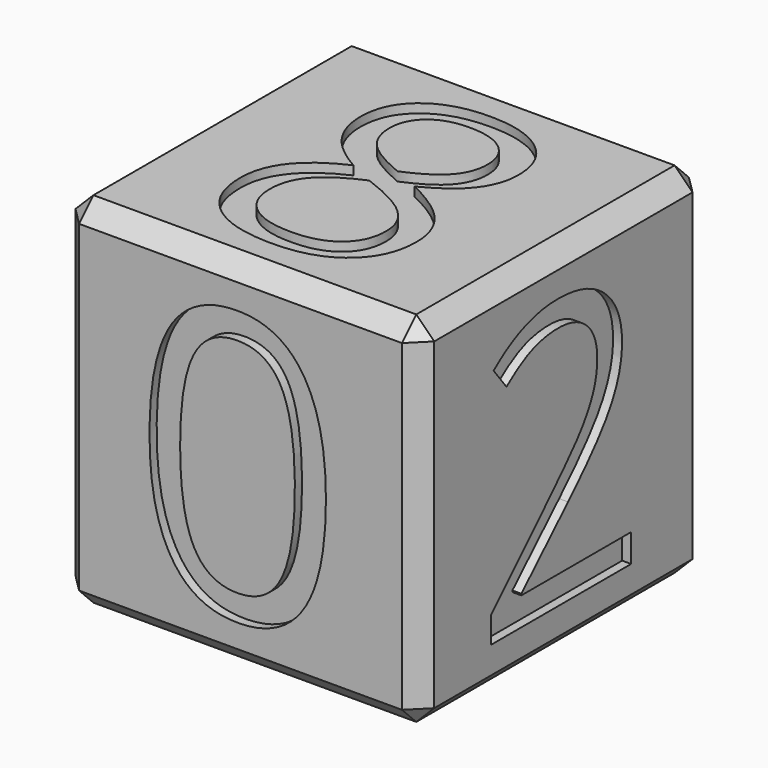
from build123d import *

# Parameters (mm, degrees)
F0_W          = 50.8
F0_H          = 50.8
F1_DEPTH      = 25.4
F1_DEPTH_BACK = 25.4
F2_SIZE       = 2.54
F3_TEXT_SIZE  = 52.9166666667
F4_DEPTH      = 1.27
F5_TEXT_SIZE  = 52.9166666667
F6_DEPTH      = 1.27
F7_TEXT_SIZE  = 52.9166666667
F8_DEPTH      = 1.27
F9_TEXT_SIZE  = 52.9166666667
F10_DEPTH     = 1.27
F11_TEXT_SIZE = 52.9166666667
F12_DEPTH     = 1.27
F13_TEXT_SIZE = 52.9166666667
F14_DEPTH     = 1.27


# Not quite as in the source:
# - Text() gives the source's letters only with a copy of the font that has no kerning and outlines rounded to 1/6400 em; it was checked with that copy


with BuildPart() as f1:
    # F0 (on Top) → F1 (new body, two sides)
    with BuildSketch(Plane.XY) as f1_sk:
        Rectangle(F0_W, F0_H)
    extrude(amount=F1_DEPTH)
    extrude(f1_sk.sketch, amount=-F1_DEPTH_BACK)

    # F2
    f2_edges = [f1.edges().sort_by_distance(p)[0] for p in [
        (0, 25.4, 25.4),
        (-25.4, 25.4, 0),
        (0, 25.4, -25.4),
        (25.4, 25.4, 0),
        (25.4, 0, 25.4),
        (-25.4, 0, 25.4),
        (0, -25.4, 25.4),
        (25.4, -25.4, 0),
        (25.4, 0, -25.4),
        (-25.4, 0, -25.4),
        (0, -25.4, -25.4),
        (-25.4, -25.4, 0),
    ]]
    chamfer(f2_edges, length=F2_SIZE)

    # F3 (on face) → F4 (cut)
    with BuildSketch(Plane.XZ.offset(25.4)):
        with Locations((-15.527734375, -19.05)):
            Text('0', F3_TEXT_SIZE, font='Open Sans', text_align=(TextAlign.LEFT, TextAlign.BOTTOM))
    extrude(amount=-F4_DEPTH, mode=Mode.SUBTRACT)

    # F5 (on face) → F6 (cut)
    with BuildSketch(Plane(origin=(-25.4, 0, 0), x_dir=(0, -1, 0), z_dir=(-1, 0, 0))):
        with Locations((-10.9512695313, -19.05)):
            Text('1', F5_TEXT_SIZE, font='Open Sans', text_align=(TextAlign.LEFT, TextAlign.BOTTOM))
    extrude(amount=-F6_DEPTH, mode=Mode.SUBTRACT)

    # F7 (on face) → F8 (cut)
    with BuildSketch(Plane.YZ.offset(25.4)):
        with Locations((-15.4243815104, -19.05)):
            Text('2', F7_TEXT_SIZE, font='Open Sans', text_align=(TextAlign.LEFT, TextAlign.BOTTOM))
    extrude(amount=-F8_DEPTH, mode=Mode.SUBTRACT)

    # F9 (on face) → F10 (cut)
    with BuildSketch(Plane(origin=(0, 0, -25.4), x_dir=(1, 0, 0), z_dir=(0, 0, -1))):
        with Locations((-15.5525390625, -19.05)):
            Text('6', F9_TEXT_SIZE, font='Open Sans', text_align=(TextAlign.LEFT, TextAlign.BOTTOM))
    extrude(amount=-F10_DEPTH, mode=Mode.SUBTRACT)

    # F11 (on face) → F12 (cut)
    with BuildSketch(Plane(origin=(0, 25.4, 0), x_dir=(-1, 0, 0), z_dir=(0, 1, 0))):
        with Locations((-15.4987955729, -19.05)):
            Text('7', F11_TEXT_SIZE, font='Open Sans', text_align=(TextAlign.LEFT, TextAlign.BOTTOM))
    extrude(amount=-F12_DEPTH, mode=Mode.SUBTRACT)

    # F13 (on face) → F14 (cut)
    with BuildSketch(Plane.XY.offset(25.4)):
        with Locations((-15.4739908854, -19.05)):
            Text('8', F13_TEXT_SIZE, font='Open Sans', text_align=(TextAlign.LEFT, TextAlign.BOTTOM))
    extrude(amount=-F14_DEPTH, mode=Mode.SUBTRACT)


solid = f1.part
